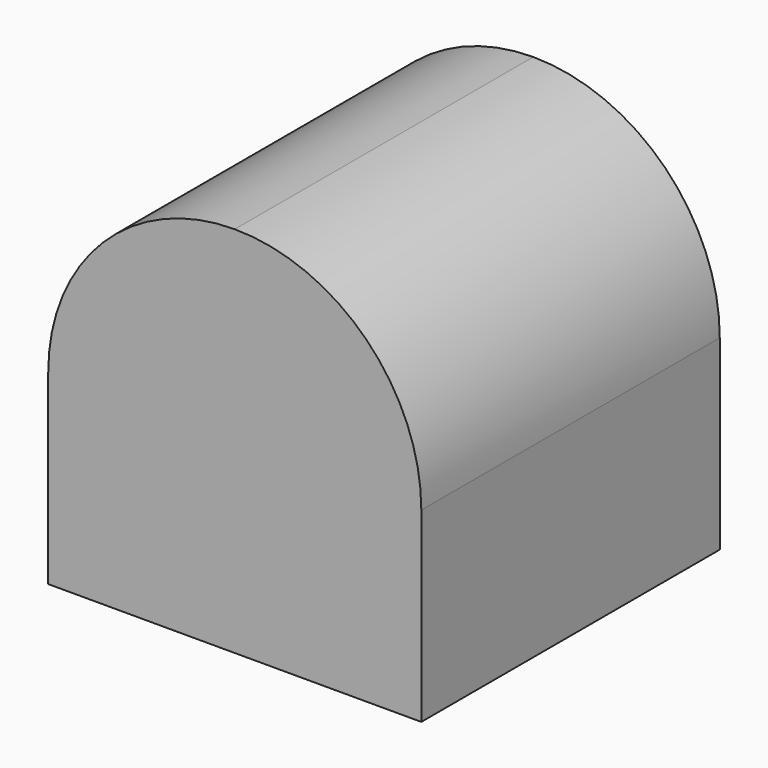
from build123d import *

# Parameters (mm, degrees)
F0_W     = 50.8
F0_H     = 50.8
F1_DEPTH = 50.8
F3_R     = 25.39999
F2_R     = 23.495
F4_DEPTH = 45.72


# Not quite as in the source:
# - a fillet or chamfer is up to 0.001 mm smaller than in the source, because OpenCascade refuses the exact size


with BuildPart() as f1:
    # F0 (on Top) → F1 (new body)
    with BuildSketch(Plane.XY):
        with Locations((-25.4, 25.4)):
            Rectangle(F0_W, F0_H)
    extrude(amount=F1_DEPTH)

    # F3 (radius 25.4 in the source; OpenCascade refuses exactly that, so slightly less here)
    f3_edges = [f1.edges().sort_by_distance(p)[0] for p in [
        (0, 25.4, 50.8),
        (-50.8, 25.4, 50.8),
    ]]
    fillet(f3_edges, radius=F3_R)

    # F2 (on face) → F4 (cut)
    with BuildSketch(Plane(origin=(0, 50.8, 0), x_dir=(-1, 0, 0), z_dir=(0, 1, 0))):
        with Locations((25.4, 24.765)):
            Circle(F2_R)
    extrude(amount=-F4_DEPTH, mode=Mode.SUBTRACT)


solid = f1.part
